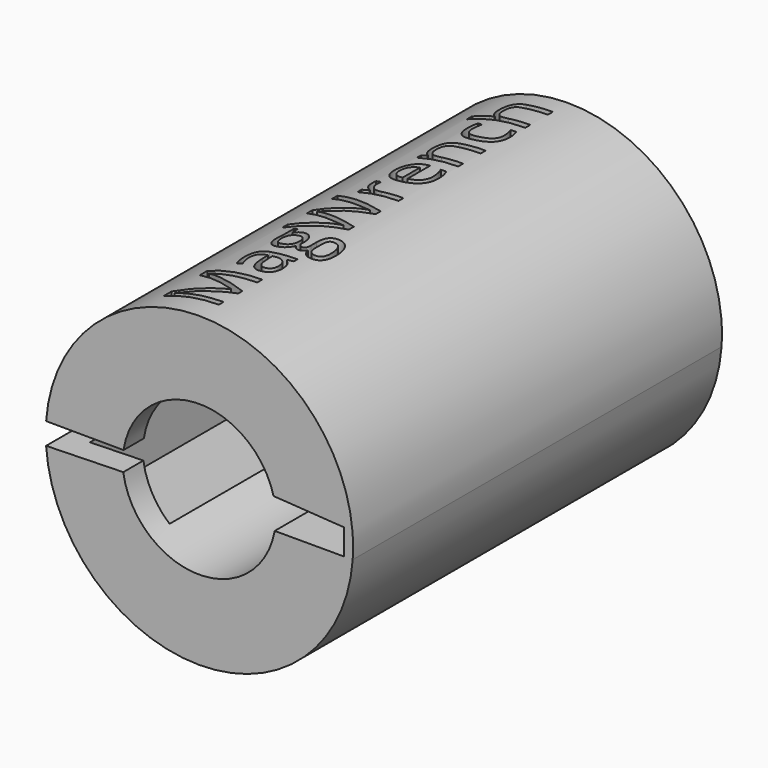
from build123d import *

# Parameters (mm, degrees)
F1_DEPTH      = 9.525
F3_W          = 2.2304863669
F3_H          = 17.0254549012
F4_DEPTH      = 2
F6_W          = 2.2374354303
F6_H          = 17.035830766
F7_DEPTH      = 2
F8_DEPTH      = 1
F9_DEPTH      = 1
F12_TEXT_SIZE = 3.1791063264
F13_DEPTH     = 1.55


# Not quite as in the source:
# - Text() gives the source's letters only with a copy of the font that has no kerning and outlines rounded to 1/6400 em; it was checked with that copy


with BuildPart() as f1:
    # F0 (on Front) → F1 (new body, symmetric)
    with BuildSketch(Plane.XZ):
        with BuildLine():
            ThreePointArc((-3.1337869048, 0.4487399592), (-0.1737428399, 3.1430183246), (3.0654538423, 0.7917204639))
            Line((3.0654538423, 0.7917204639), (5.9831817634, 0.6017680259))
            Line((5.9831817634, 0.6017680259), (5.9831817634, -0.4601007677))
            Line((5.9831817634, -0.4601007677), (3.1110077623, -0.4601007677))
            ThreePointArc((3.1110077623, -0.4601007677), (-0.0609427481, -3.0658926252), (-3.1454691198, -0.3571810666))
            Line((-3.1454691198, -0.3571810666), (-6.3349851864, -0.4364203109))
            ThreePointArc((-6.3349851864, -0.4364203109), (-0.0118698407, -6.349988906), (6.3333093469, -0.4601007677))
            ThreePointArc((6.3333093469, -0.4601007677), (6.3497169322, 0.0599573295), (6.3234918301, 0.5796128666))
            ThreePointArc((6.3234918301, 0.5796128666), (-0.0589289492, 6.3497265594), (-6.3331599818, 0.4621521879))
            Line((-6.3331599818, 0.4621521879), (-3.1337869048, 0.4487399592))
        make_face()
    extrude(amount=F1_DEPTH, both=True)

    # F3 (on offset) → F4 (cut)
    with BuildSketch(Plane(origin=(0.0018260765, 0, 0.435595022), x_dir=(0.9999912131, 0, -0.0041921059), z_dir=(-0.0041921059, 0, -0.9999912131))):
        with Locations((-4.2508837173, -0.0363742001)):
            Rectangle(F3_W, F3_H)
    extrude(amount=-F4_DEPTH, mode=Mode.SUBTRACT)

    # F6 (on offset) → F7 (cut)
    with BuildSketch(Plane(origin=(0.0069280015, 0, -0.2788639928), x_dir=(0.9996915391, 0, 0.024835994), z_dir=(-0.024835994, 0, 0.9996915391))):
        with Locations((-4.2403930663, 0.0314759091)):
            Rectangle(F6_W, F6_H)
    extrude(amount=-F7_DEPTH, mode=Mode.SUBTRACT)

    # F8 (cut): a face of the model
    f8_faces = [f1.faces().sort_by_distance(p)[0] for p in [
        (-3.0864096747, 0.0314759091, -1.4582751573),
    ]]
    extrude(f8_faces, amount=-F8_DEPTH, mode=Mode.SUBTRACT)

    # F9 (cut): a face of the model
    f9_faces = [f1.faces().sort_by_distance(p)[0] for p in [
        (-3.1295947988, 0.0363742001, 1.4487311723),
    ]]
    extrude(f9_faces, amount=-F9_DEPTH, mode=Mode.SUBTRACT)

    # F12 (on plane+point) → F13 (cut)
    with BuildSketch(Plane.XY.offset(6.35)):
        with Locations(Location((0, -8.836467237), (0, 0, 90))):
            Text('MagWrench', F12_TEXT_SIZE, font='Open Sans', text_align=(TextAlign.LEFT, TextAlign.BOTTOM))
    extrude(amount=-F13_DEPTH, mode=Mode.SUBTRACT)


solid = f1.part
